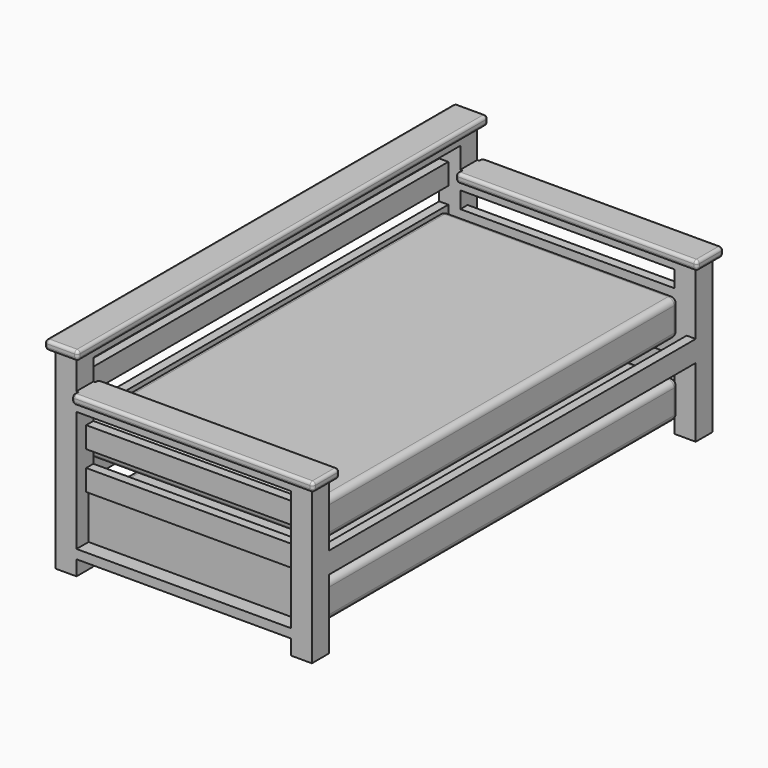
from build123d import *

# Parameters (mm, degrees)
F0_W           = 901.7
F0_H           = 508
F1_DEPTH       = 88.9
F2_W           = 901.7
F2_H           = 88.9
F3_DEPTH       = 38.1
F5_START       = 12.7
F4_W           = 901.7
F4_H           = 190.5
F5_DEPTH       = 12.7
F6_W           = 88.9
F6_H           = 38.1
F6_W_2         = 38.1
F6_H_2         = 88.9
F7_DEPTH       = 965.2
F9_START       = 76.2
F9_DEPTH       = 863.6
F10_W          = 139.7
F10_H          = 38.1
F11_DEPTH      = 1016
F13_DEPTH      = 25.4
F13_DEPTH_BACK = 1054.1
F16_START      = 25.4
F15_W          = 990.6
F15_H          = 152.4
F16_DEPTH      = 1879.6
F17_R          = 25.4
F19_R          = 12.7


# Not quite as in the source:
# - a feature names something its author has since deleted; it is built from what else it names


with BuildPart() as f1:
    # F0 (on Front) → F1 (new body)
    with BuildSketch(Plane.XZ):
        Polygon((1079.5, 647.7), (88.9, 647.7), (88.9, 812.8), (0, 812.8), (0, 0), (88.9, 0), (88.9, 63.5), (990.6, 63.5), (990.6, 0), (1079.5, 0), align=None)
        with Locations((539.75, 355.6)):
            Rectangle(F0_W, F0_H, mode=Mode.SUBTRACT)
    extrude(amount=F1_DEPTH)

    # F2 (on Front) → F3 (join)
    with BuildSketch(Plane.XZ):
        with Locations((539.75, 495.3)):
            Rectangle(F2_W, F2_H)
        with Locations((539.75, 336.55)):
            Rectangle(F2_W, F2_H)
    extrude(amount=F3_DEPTH)

    # F4 (on Front) → F5 (join)
    with BuildSketch(Plane.XZ.offset(F5_START)):
        with Locations((539.75, 196.85)):
            Rectangle(F4_W, F4_H)
    extrude(amount=F5_DEPTH)

    # F6 (on Front) → F7 (join)
    with BuildSketch(Plane.XZ):
        with Locations((44.45, 793.75)):
            Rectangle(F6_W, F6_H)
        with Locations((19.05, 654.05)):
            Rectangle(F6_W_2, F6_H_2)
        with Locations((19.05, 495.3)):
            Rectangle(F6_W_2, F6_H_2)
        with Locations((19.05, 336.55)):
            Rectangle(F6_W_2, F6_H_2)
        with Locations((1060.45, 336.55)):
            Rectangle(F6_W_2, F6_H_2)
    extrude(amount=-F7_DEPTH)

    # F10 (on face) → F11 (join)
    with BuildSketch(Plane.YZ.offset(88.9)):
        with Locations((-44.45, 666.75)):
            Rectangle(F10_W, F10_H)
    extrude(amount=F11_DEPTH)

    # F12 (on face) → F13 (join, two sides)
    with BuildSketch(Plane.XZ.offset(88.9)) as f13_sk:
        Polygon((114.3, 850.9), (-25.4, 850.9), (-25.4, 812.8), (0, 812.8), (88.9, 812.8), (114.3, 812.8), align=None)
    extrude(amount=F13_DEPTH)
    extrude(f13_sk.sketch, amount=-F13_DEPTH_BACK)

    # F14: F1, F9 across face


with BuildPart() as f9:
    # F8 (on face) → F9 (new body)
    with BuildSketch(Plane(origin=(0, 0, 0), x_dir=(-1, 0, 0), z_dir=(0, 1, 0)).offset(F9_START)):
        Polygon((-990.6, 381), (-965.2, 381), (-114.3, 381), (-88.9, 381), (-88.9, 450.85), (-990.6, 450.85), align=None)
    extrude(amount=F9_DEPTH)


with BuildPart() as f1_1:
    add(f1.part)
    add(f1.part.mirror(Plane(origin=(44.45, 965.2, 817.0333333333), x_dir=(1, 0, 0), z_dir=(0, 1, 0))))
    add(f9.part.mirror(Plane(origin=(44.45, 965.2, 817.0333333333), x_dir=(1, 0, 0), z_dir=(0, 1, 0))))

    # F19
    f19_edges = [f1_1.edges().sort_by_distance(p)[0] for p in [
        (44.45, -114.3, 850.9),
        (-25.4, -114.3, 831.85),
        (44.45, -114.3, 812.8),
        (114.3, -114.3, 831.85),
        (114.3, 965.2, 812.8),
        (114.3, 965.2, 850.9),
        (114.3, 2044.7, 831.85),
        (596.9, -114.3, 685.8),
        (596.9, -114.3, 647.7),
        (88.9, -114.3, 666.75),
        (1104.9, -114.3, 666.75),
        (1104.9, -44.45, 685.8),
        (1104.9, -44.45, 647.7),
        (1104.9, 25.4, 666.75),
        (596.9, 25.4, 647.7),
        (596.9, 25.4, 685.8),
        (88.9, 25.4, 666.75),
        (596.9, 2044.7, 685.8),
        (596.9, 2044.7, 647.7),
        (88.9, 2044.7, 666.75),
        (1104.9, 2044.7, 666.75),
        (1104.9, 1974.85, 685.8),
        (1104.9, 1974.85, 647.7),
        (1104.9, 1905, 666.75),
        (44.45, 2044.7, 850.9),
        (-25.4, 2044.7, 831.85),
        (44.45, 2044.7, 812.8),
        (596.9, 1905, 647.7),
        (596.9, 1905, 685.8),
        (88.9, 1905, 666.75),
        (-25.4, 965.2, 812.8),
        (-25.4, 965.2, 850.9),
        (88.9, -101.6, 685.8),
        (88.9, -101.6, 647.7),
        (88.9, 12.7, 685.8),
        (88.9, 2032, 685.8),
        (88.9, 2032, 647.7),
        (88.9, 1917.7, 685.8),
        (88.9, 1917.7, 647.7),
        (88.9, 12.7, 647.7),
    ]]
    fillet(f19_edges, radius=F19_R)


with BuildPart() as f16:
    # F15 (on face) → F16 (new body)
    with BuildSketch(Plane(origin=(0, 0, 0), x_dir=(-1, 0, 0), z_dir=(0, 1, 0)).offset(F16_START)):
        with Locations((-533.4, 457.2)):
            Rectangle(F15_W, F15_H)
    extrude(amount=F16_DEPTH)

    # F17
    f17_edges = [f16.edges().sort_by_distance(p)[0] for p in [
        (38.1, 965.2, 533.4),
        (1028.7, 965.2, 533.4),
        (533.4, 25.4, 533.4),
        (533.4, 1905, 533.4),
        (1028.7, 965.2, 381),
        (38.1, 965.2, 381),
        (533.4, 25.4, 381),
        (533.4, 1905, 381),
        (1028.7, 25.4, 457.2),
        (1028.7, 1905, 457.2),
        (38.1, 25.4, 457.2),
        (38.1, 1905, 457.2),
    ]]
    fillet(f17_edges, radius=F17_R)


with BuildPart() as f18_1:
    # F18: copy of F16
    add(f16.part.moved(Location((0, 0, -304.8))))


solid = Compound([f9.part, f1_1.part, f16.part, f18_1.part])
